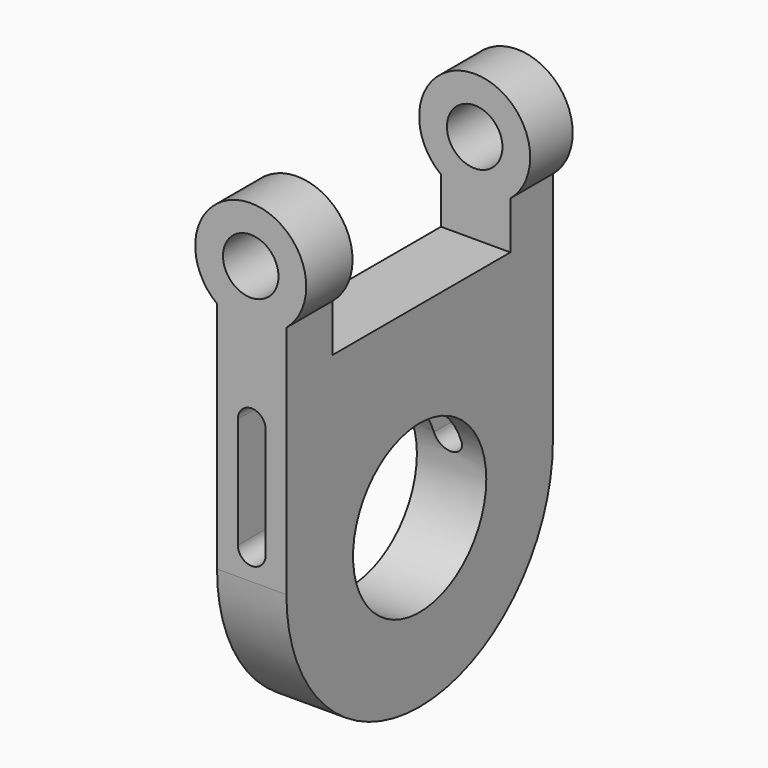
from build123d import *

# Parameters (mm, degrees)
F0_R     = 12.7
F1_DEPTH = 152.4
F2_R     = 76.19999
F3_R     = 38.1
F4_DEPTH = 41.7364233324
F7_DEPTH = 96.9898923586
F8_DEPTH = 152.401


# Not quite as in the source:
# - a fillet or chamfer is up to 0.001 mm smaller than in the source, because OpenCascade refuses the exact size


with BuildPart() as f1:
    # F0 (on Front) → F1 (new body)
    with BuildSketch(Plane.XZ):
        with BuildLine():
            Line((-39.075684309, -141.72433921), (-39.075684309, 42.0253665879))
            ThreePointArc((-39.075684309, 42.0253665879), (-56.0010235987, 86.8688094558), (-70.825684309, 41.2877726846))
            Line((-70.825684309, 41.2877726846), (-70.825684309, -141.72433921))
            Line((-70.825684309, -141.72433921), (-39.075684309, -141.72433921))
        make_face()
        with Locations((-55.4111076414, 61.47566079)):
            Circle(F0_R, mode=Mode.SUBTRACT)
        with BuildLine():
            Line((-61.300684309, -52.82433921), (-61.300684309, -2.02433921))
            ThreePointArc((-61.300684309, -2.02433921), (-54.950684309, 4.32566079), (-48.600684309, -2.02433921))
            Line((-48.600684309, -2.02433921), (-48.600684309, -52.82433921))
            ThreePointArc((-48.600684309, -52.82433921), (-54.950684309, -59.17433921), (-61.300684309, -52.82433921))
        make_face(mode=Mode.SUBTRACT)
        with BuildLine():
            ThreePointArc((-48.600684309, -2.02433921), (-54.950684309, 4.32566079), (-61.300684309, -2.02433921))
            Line((-61.300684309, -2.02433921), (-61.300684309, -52.82433921))
            ThreePointArc((-61.300684309, -52.82433921), (-54.950684309, -59.17433921), (-48.600684309, -52.82433921))
            Line((-48.600684309, -52.82433921), (-48.600684309, -2.02433921))
        make_face()
    extrude(amount=F1_DEPTH)

    # F2 (radius 76.2 in the source; OpenCascade refuses exactly that, so slightly less here)
    f2_edges = [f1.edges().sort_by_distance(p)[0] for p in [
        (-54.950684, 0, -141.724339),
        (-54.950684, -152.4, -141.724339),
    ]]
    fillet(f2_edges, radius=F2_R)

    # F3 (on face) → F4 (cut, through all)
    with BuildSketch(Plane.YZ.offset(-39.075684309)):
        with Locations((-76.2, -65.52433921)):
            Circle(F3_R)
    extrude(amount=-F4_DEPTH, mode=Mode.SUBTRACT)

    # F6 (on offset) → F7 (cut, through all)
    with BuildSketch(Plane.YZ.offset(-127)):
        Polygon((-24.3093731642, 100.3912016645), (-125.9093731642, 96.466931504), (-125.9093731642, 20.266931504), (-24.3093731642, 20.266931504), align=None)
    extrude(amount=F7_DEPTH, mode=Mode.SUBTRACT)

    # F0 (on Front) → F8 (cut, through all)
    with BuildSketch(Plane.XZ):
        with BuildLine():
            ThreePointArc((-48.600684309, -2.02433921), (-54.950684309, 4.32566079), (-61.300684309, -2.02433921))
            Line((-61.300684309, -2.02433921), (-61.300684309, -52.82433921))
            ThreePointArc((-61.300684309, -52.82433921), (-54.950684309, -59.17433921), (-48.600684309, -52.82433921))
            Line((-48.600684309, -52.82433921), (-48.600684309, -2.02433921))
        make_face()
    extrude(amount=F8_DEPTH, mode=Mode.SUBTRACT)


solid = f1.part
